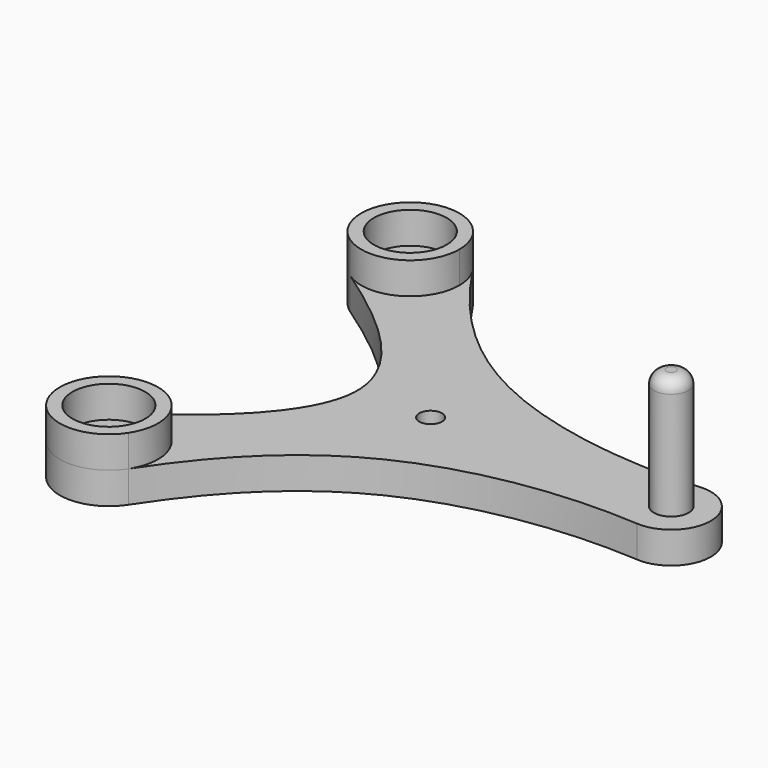
from build123d import *

# Parameters (mm, degrees)
F0_R     = 1.8
F0_R_2   = 2.75
F0_R_3   = 5.75
F1_DEPTH = 5
F2_DEPTH = 5
F3_DEPTH = 19
F4_R     = 2


with BuildPart() as f1:
    # F0 (on Top) → F1 (new body)
    with BuildSketch(Plane.XY):
        with BuildLine():
            ThreePointArc((-20.5278924674, 33.9874824942), (-19.5887790687, 31.9605740028), (-19.2668247456, 29.75))
            ThreePointArc((-19.2668247456, 29.75), (-23.4010274534, 22.8951834494), (-31.3928918273, 23.3537091298))
            add(Edge.make_bspline(
                [(-31.3928918273, 23.3537091298), (-21.6948142815, 16.7187016285), (-1.5034517677, 0.3606813033), (-21.4654354866, -17.2386169061), (-31.0762132171, -23.1481922751)],
                knots=[0, 0, 0, 0, 0.5014830117, 1, 1, 1, 1], degree=3))
            ThreePointArc((-31.0762132171, -23.1481922751), (-23.2351426235, -22.9852841651), (-19.2668247456, -29.75))
            ThreePointArc((-19.2668247456, -29.75), (-19.5887790687, -31.9605740028), (-20.5278924674, -33.9874824942))
            add(Edge.make_bspline(
                [(-20.5278924674, -33.9874824942), (-14.2038261776, -24.3033273542), (0.8934932617, -9.0476289983), (25.586991994, -5.4412595008), (37.5868020457, -6.2363264387)],
                knots=[0, 0, 0, 0, 0.4873954252, 1, 1, 1, 1], degree=3))
            ThreePointArc((37.5868020457, -6.2363264387), (44.25, 0), (37.5868020457, 6.2363264387))
            add(Edge.make_bspline(
                [(-20.5278924674, 33.9874824942), (-14.2038261776, 24.3033273542), (0.8934932617, 9.0476289983), (25.586991994, 5.4412595008), (37.5868020457, 6.2363264387)],
                knots=[0, 0, 0, 0, 0.4873954252, 1, 1, 1, 1], degree=3))
        make_face()
        Circle(F0_R, mode=Mode.SUBTRACT)
        with Locations((38, 0)):
            Circle(F0_R_2, mode=Mode.SUBTRACT)
        with BuildLine():
            ThreePointArc((-31.3928918273, 23.3537091298), (-23.4010274534, 22.8951834494), (-19.2668247456, 29.75))
            ThreePointArc((-19.2668247456, 29.75), (-19.5887790687, 31.9605740028), (-20.5278924674, 33.9874824942))
            ThreePointArc((-20.5278924674, 33.9874824942), (-32.4376488366, 35.2886971549), (-31.3928918273, 23.3537091298))
        make_face()
        with Locations((-27.0168247456, 29.75)):
            Circle(F0_R_3, mode=Mode.SUBTRACT)
        with BuildLine():
            ThreePointArc((-19.2668247456, -29.75), (-23.2351426235, -22.9852841651), (-31.0762132171, -23.1481922751))
            ThreePointArc((-31.0762132171, -23.1481922751), (-32.5709424875, -35.1550232293), (-20.5278924674, -33.9874824942))
            ThreePointArc((-20.5278924674, -33.9874824942), (-19.5887790687, -31.9605740028), (-19.2668247456, -29.75))
        make_face()
        with Locations((-27.0168247456, -29.75)):
            Circle(F0_R_3, mode=Mode.SUBTRACT)
        with Locations((-27.0168247456, 29.75)):
            Circle(F0_R_3)
        with Locations((-27.0168247456, -29.75)):
            Circle(F0_R_3)
        with Locations((38, 0)):
            Circle(F0_R_2)
    extrude(amount=-F1_DEPTH)

    # F0 (on Top) → F2 (join)
    with BuildSketch(Plane.XY):
        with BuildLine():
            ThreePointArc((-31.3928918273, 23.3537091298), (-23.4010274534, 22.8951834494), (-19.2668247456, 29.75))
            ThreePointArc((-19.2668247456, 29.75), (-19.5887790687, 31.9605740028), (-20.5278924674, 33.9874824942))
            ThreePointArc((-20.5278924674, 33.9874824942), (-32.4376488366, 35.2886971549), (-31.3928918273, 23.3537091298))
        make_face()
        with Locations((-27.0168247456, 29.75)):
            Circle(F0_R_3, mode=Mode.SUBTRACT)
        with BuildLine():
            ThreePointArc((-19.2668247456, -29.75), (-23.2351426235, -22.9852841651), (-31.0762132171, -23.1481922751))
            ThreePointArc((-31.0762132171, -23.1481922751), (-32.5709424875, -35.1550232293), (-20.5278924674, -33.9874824942))
            ThreePointArc((-20.5278924674, -33.9874824942), (-19.5887790687, -31.9605740028), (-19.2668247456, -29.75))
        make_face()
        with Locations((-27.0168247456, -29.75)):
            Circle(F0_R_3, mode=Mode.SUBTRACT)
    extrude(amount=F2_DEPTH)

    # F0 (on Top) → F3 (join)
    with BuildSketch(Plane.XY):
        with Locations((38, 0)):
            Circle(F0_R_2)
    extrude(amount=F3_DEPTH)

    # F4
    f4_edges = [f1.edges().sort_by_distance(p)[0] for p in [
        (35.25, 0, 19),
    ]]
    fillet(f4_edges, radius=F4_R)


solid = f1.part
